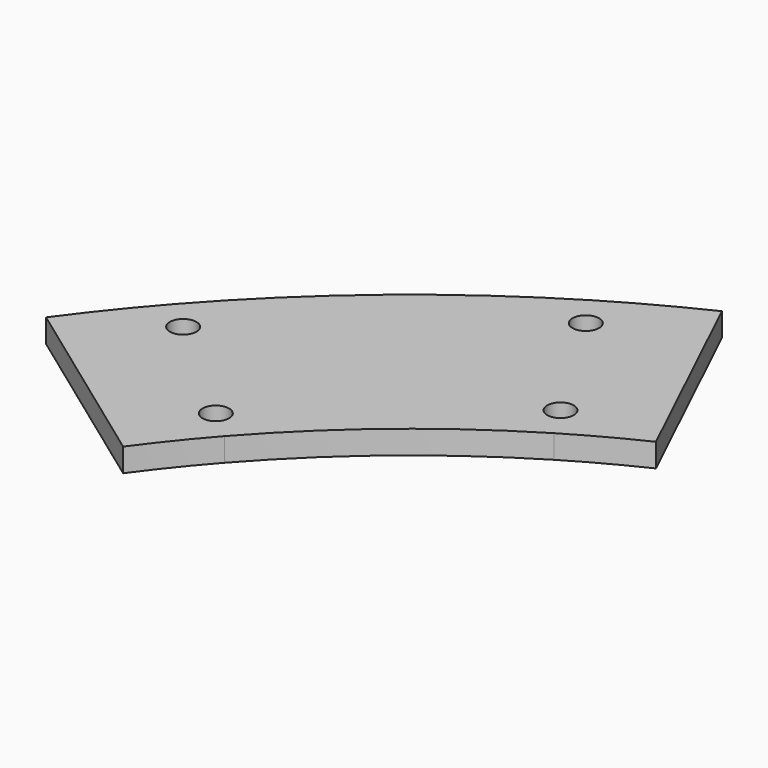
from build123d import *

# Parameters (mm, degrees)
F1_DEPTH = 3
F2_D     = 3.4


with BuildPart() as f1:
    # F0 (on Top) → F1 (new body)
    with BuildSketch(Plane.XY):
        with BuildLine():
            ThreePointArc((-55.6590960491, 92.5530389939), (-51.154476682, 95.1168729269), (-46.5320369414, 97.4616311072))
            Line((-46.5320369414, 97.4616311072), (-59.0267505646, 123.6318839045))
            ThreePointArc((-59.0267505646, 123.6318839045), (-64.8904009762, 120.6575147314), (-70.6045940623, 117.4052439089))
            ThreePointArc((-70.6045940623, 117.4052439089), (-87.6662762423, 105.278791833), (-102.6814380892, 90.6946650688))
            ThreePointArc((-102.6814380892, 90.6946650688), (-106.9145490542, 85.6637566334), (-110.9014115399, 80.4355451181))
            Line((-110.9014115399, 80.4355451181), (-87.4259302651, 63.4090428669))
            ThreePointArc((-87.4259302651, 63.4090428669), (-84.2830021741, 67.5305526745), (-80.9459511944, 71.4965242878))
            ThreePointArc((-80.9459511944, 71.4965242878), (-69.1091812713, 82.9935001311), (-55.6590960491, 92.5530389939))
        make_face()
    extrude(amount=F1_DEPTH)

    # F2 (through all)
    with Locations(Plane(origin=(0, 0, 0), x_dir=(1, 0, 0), z_dir=(0, 0, -1))):
        with Locations((-98.9339403487, -87.3846407962), (-84.6934489349, -74.8065485604), (-58.2359060514, -96.8379019102), (-68.02778406, -113.1203809925)):
            Hole(F2_D / 2)


solid = f1.part
